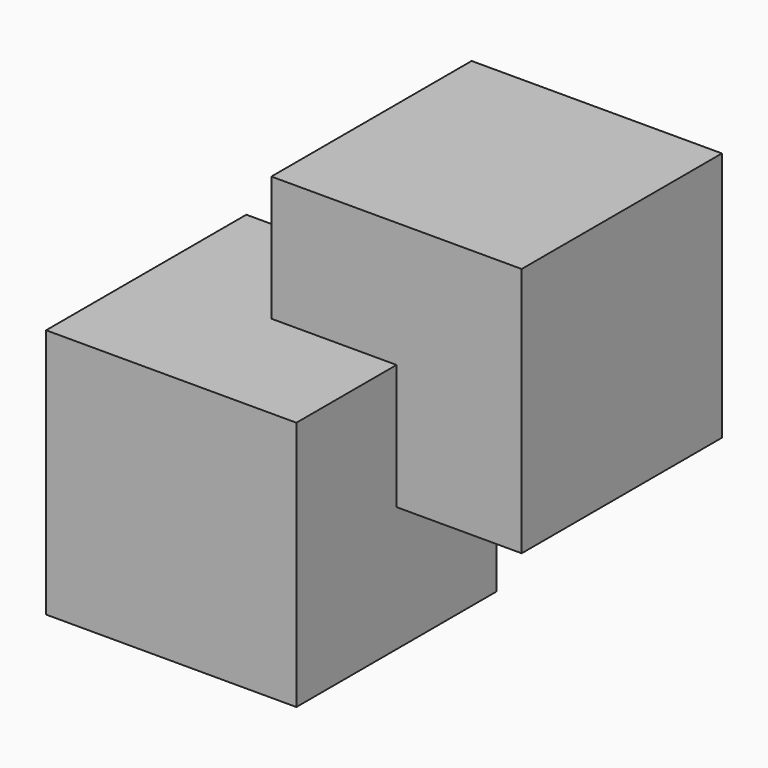
from build123d import *

# Parameters (mm, degrees)
F0_W            = 40
F0_H            = 40
F1_DEPTH        = 20
F1_COPIES_COUNT = 2
F1_COPIES_PITCH = 34.641016


# Not quite as in the source:
# - a pattern or mirror of a feature is missing from the dataset's text; its kind, count and spacing are read off the source's solid


with BuildPart() as f1:
    # F0 (on Top) → F1 (new body, symmetric)
    with BuildSketch(Plane.XY):
        Rectangle(F0_W, F0_H)
    extrude(amount=F1_DEPTH, both=True)


with BuildPart() as f1_copies_1:
    # F1_copies: instance of F1
    add(f1.part.moved(Location(Vector(0.5773502692, 0.5773502692, 0.5773502692) * (1 * F1_COPIES_PITCH))))


with BuildPart() as f2_1:
    # F2: copy of F1
    add(f1.part.moved(Location((20, 20, 20))))

    # F3: intersect F1
    add(f1.part, mode=Mode.INTERSECT)


solid = Compound([f1.part, f1_copies_1.part, f2_1.part])
